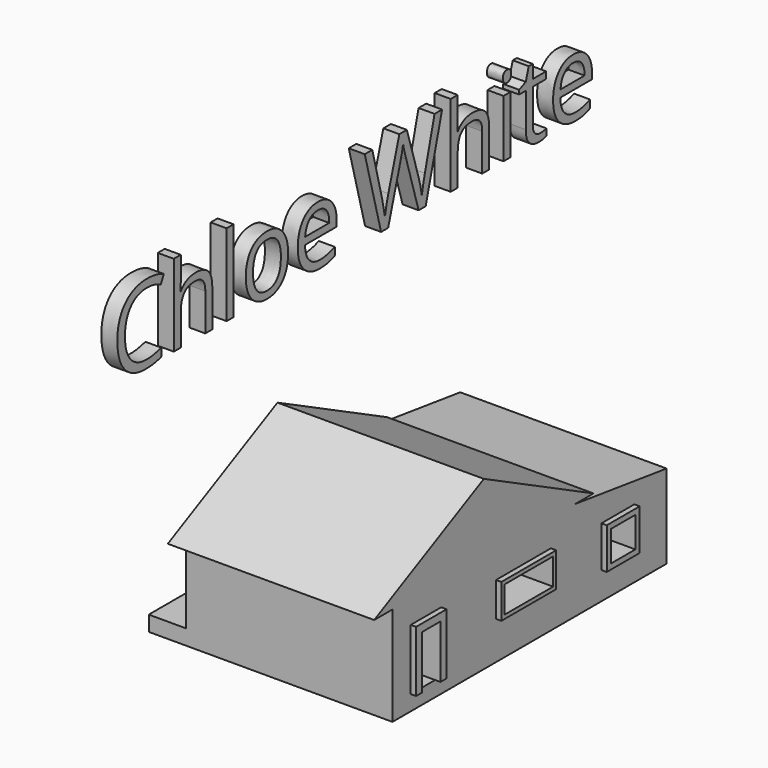
from build123d import *

# Parameters (mm, degrees)
F0_W         = 228.6
F0_H         = 114.3
F0_W_2       = 381
F0_H_2       = 50.8
F0_W_3       = 137.16
F0_H_3       = 137.16
F1_DEPTH     = 688.34
F0_W_4       = 203.2
F0_H_4       = 88.9
F0_W_5       = 101.6
F0_H_5       = 101.6
F2_DEPTH     = 706.12
F3_DEPTH     = 124.46
F4_TEXT_SIZE = 358.8063021501
F5_DEPTH     = 53.34


# Not quite as in the source:
# - Text() gives the source's letters only with a copy of the font that has no kerning and outlines rounded to 1/6400 em; it was checked with that copy


with BuildPart() as f1:
    # F0 (on Right) → F1 (new body)
    with BuildSketch(Plane.YZ):
        Polygon((381, 0), (0, 0), (-381, 0), (-381, -279.4), (-304.8, -279.4), (-304.8, -76.2), (-177.8, -76.2), (-177.8, -279.4), (381, -279.4), (381, -50.8), align=None)
        with Locations((165.1, -146.05)):
            Rectangle(F0_W, F0_H, mode=Mode.SUBTRACT)
        Polygon((-304.8, -279.4), (-381, -279.4), (-381, -330.2), (381, -330.2), (381, -279.4), (-177.8, -279.4), (-203.2, -279.4), (-279.4, -279.4), align=None)
        with Locations((571.5, -304.8)):
            Rectangle(F0_W_2, F0_H_2)
        Polygon((762, -101.6), (381, -50.8), (381, -279.4), (762, -279.4), align=None)
        with Locations((558.8, -169.7828996188)):
            Rectangle(F0_W_3, F0_H_3, mode=Mode.SUBTRACT)
        Polygon((762, -50.8), (381, 0), (381, -50.8), (762, -101.6), align=None)
        Polygon((0, 190.5), (381, 0), (457.2, 0), (0, 228.6), align=None)
        Polygon((0, 190.5), (0, 0), (381, 0), align=None)
        Polygon((-381, 0), (0, 0), (0, 190.5), align=None)
        Polygon((-457.2, 0), (-381, 0), (0, 190.5), (0, 228.6), align=None)
    extrude(amount=F1_DEPTH)

    # F0 (on Right) → F2 (join)
    with BuildSketch(Plane.YZ):
        Polygon((-304.8, -76.2), (-304.8, -279.4), (-279.4, -279.4), (-279.4, -101.6), (-203.2, -101.6), (-203.2, -279.4), (-177.8, -279.4), (-177.8, -76.2), align=None)
        with Locations((165.1, -146.05)):
            Rectangle(F0_W, F0_H)
        with Locations((165.1, -146.05)):
            Rectangle(F0_W_4, F0_H_4, mode=Mode.SUBTRACT)
        with Locations((558.8, -169.7828996188)):
            Rectangle(F0_W_3, F0_H_3)
        with Locations((558.8, -169.7828996188)):
            Rectangle(F0_W_5, F0_H_5, mode=Mode.SUBTRACT)
    extrude(amount=F2_DEPTH)

    # F0 (on Right) → F3 (join)
    with BuildSketch(Plane.YZ):
        Polygon((-304.8, -279.4), (-381, -279.4), (-381, -330.2), (381, -330.2), (381, -279.4), (-177.8, -279.4), (-203.2, -279.4), (-279.4, -279.4), align=None)
        with Locations((571.5, -304.8)):
            Rectangle(F0_W_2, F0_H_2)
    extrude(amount=-F3_DEPTH)


with BuildPart() as f5:
    # F4 (on face) → F5 (new body)
    with BuildSketch(Plane.YZ):
        with Locations((-756.1753988266, 598.4408259392)):
            Text('Chloe White', F4_TEXT_SIZE, font='Open Sans', text_align=(TextAlign.LEFT, TextAlign.BOTTOM))
    extrude(amount=F5_DEPTH)


solid = Compound([f1.part, f5.part])
